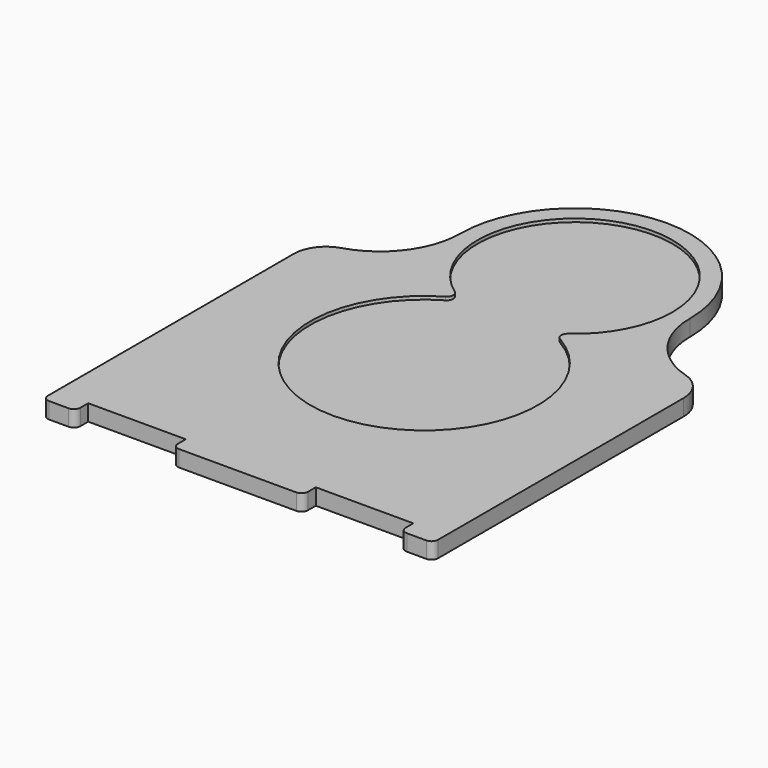
from build123d import *

# Parameters (mm, degrees)
F1_DEPTH = 6.35
F2_R     = 12.7
F3_R     = 2.54
F5_DEPTH = 1.27
F6_R     = 2.54


# Not quite as in the source:
# - a feature names something its author has since deleted; it is built from what else it names


with BuildPart() as f1:
    # F0 (on Top) → F1 (new body)
    with BuildSketch(Plane.XY):
        with BuildLine():
            Line((0, 127), (0, 0))
            Line((0, 0), (0, -6.35))
            Line((0, -6.35), (12.7, -6.35))
            Line((12.7, -6.35), (12.7, 0))
            Line((12.7, 0), (50.8, 0))
            Line((50.8, 0), (50.8, -6.35))
            Line((50.8, -6.35), (101.6, -6.35))
            Line((101.6, -6.35), (101.6, 0))
            Line((101.6, 0), (139.7, 0))
            Line((139.7, 0), (139.7, -6.35))
            Line((139.7, -6.35), (152.4, -6.35))
            Line((152.4, -6.35), (152.4, 0))
            Line((152.4, 0), (152.4, 127))
            ThreePointArc((152.4, 127), (130.249490442, 136.1750414724), (121.0744489697, 158.3255510303))
            ThreePointArc((121.0744489697, 158.3255510303), (76.2, 203.2), (31.3255510303, 158.3255510303))
            ThreePointArc((31.3255510303, 158.3255510303), (22.150509558, 136.1750414724), (0, 127))
        make_face()
    extrude(amount=F1_DEPTH)

    # F2
    f2_edges = [f1.edges().sort_by_distance(p)[0] for p in [
        (0, 127, 3.175),
        (152.4, 127, 3.175),
    ]]
    fillet(f2_edges, radius=F2_R)

    # F3
    f3_edges = [f1.edges().sort_by_distance(p)[0] for p in [
        (0, -6.35, 3.175),
        (12.7, -6.35, 3.175),
        (50.8, -6.35, 3.175),
        (101.6, -6.35, 3.175),
        (139.7, -6.35, 3.175),
        (152.4, -6.35, 3.175),
    ]]
    fillet(f3_edges, radius=F3_R)

    # F4 (on face) → F5 (cut)
    with BuildSketch(Plane.XY.offset(6.35)):
        with BuildLine():
            ThreePointArc((94.7584962883, 125.0510530549), (109.0533766041, 139.0313641932), (114.3, 158.3255510303))
            ThreePointArc((114.3, 158.3255510303), (56.9058131628, 191.1789276345), (57.6415037117, 125.0510530549))
            ThreePointArc((57.6415037117, 125.0510530549), (76.2, 129.1106492996), (94.7584962883, 125.0510530549))
        make_face()
        with BuildLine():
            ThreePointArc((94.7584962883, 125.0510530549), (76.2, 120.2255510303), (57.6415037117, 125.0510530549))
            ThreePointArc((57.6415037117, 125.0510530549), (52.2116972257, 47.2392138647), (120.65, 84.6606492996))
            ThreePointArc((120.65, 84.6606492996), (113.6214354349, 108.6489520739), (94.7584962883, 125.0510530549))
        make_face()
        with BuildLine():
            ThreePointArc((94.7584962883, 125.0510530549), (76.2, 129.1106492996), (57.6415037117, 125.0510530549))
            ThreePointArc((57.6415037117, 125.0510530549), (76.2, 120.2255510303), (94.7584962883, 125.0510530549))
        make_face()
    extrude(amount=-F5_DEPTH, mode=Mode.SUBTRACT)

    # F6
    f6_edges = [f1.edges().sort_by_distance(p)[0] for p in [
        (57.641504, 125.051053, 5.715),
        (94.758496, 125.051053, 5.715),
    ]]
    fillet(f6_edges, radius=F6_R)


solid = f1.part
